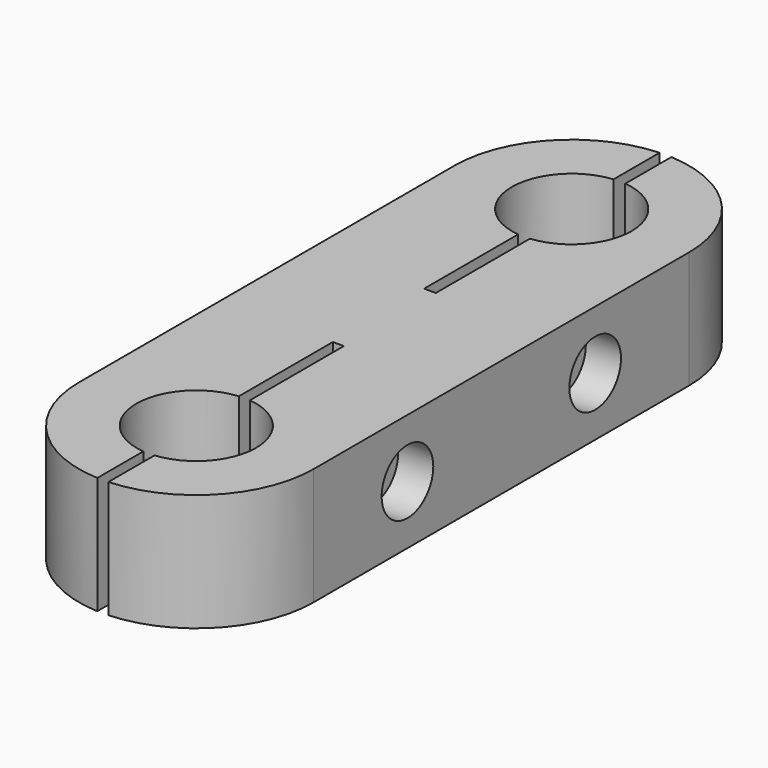
from build123d import *

# Parameters (mm, degrees)
F0_R     = 5.1
F1_DEPTH = 10
F2_R     = 1.5
F3_DEPTH = 25
F5_DEPTH = 25
F6_R     = 2.75
F6_R_2   = 1.5
F7_DEPTH = 3
F8_R     = 1.5
F9_DEPTH = 2


# Not quite as in the source:
# - a feature names something its author has since deleted; it is built from what else it names


with BuildPart() as f1:
    # F0 (on Top) → F1 (new body)
    with BuildSketch(Plane.XY):
        with BuildLine():
            ThreePointArc((-10, 0), (0, -10), (10, 0))
            ThreePointArc((10, 0), (0, 10), (-10, 0))
        make_face()
        Circle(F0_R, mode=Mode.SUBTRACT)
        with BuildLine():
            Line((10, -40), (10, 0))
            ThreePointArc((10, 0), (0, -10), (-10, 0))
            Line((-10, 0), (-10, -40))
            ThreePointArc((-10, -40), (0, -30), (10, -40))
        make_face()
        with BuildLine():
            ThreePointArc((-10, -40), (0, -50), (10, -40))
            ThreePointArc((10, -40), (0, -30), (-10, -40))
        make_face()
        with Locations((0, -40)):
            Circle(F0_R, mode=Mode.SUBTRACT)
    extrude(amount=F1_DEPTH)

    # F2 (on face) → F3 (cut)
    with BuildSketch(Plane.YZ.offset(10)):
        with Locations((-30, 5)):
            Circle(F2_R)
        with Locations((-10, 5)):
            Circle(F2_R)
    extrude(amount=-F3_DEPTH, mode=Mode.SUBTRACT)

    # F4 (on face) → F5 (cut)
    with BuildSketch(Plane.XY.offset(10)):
        with BuildLine():
            ThreePointArc((0.5, 9.9874921777), (0, 10), (-0.5, 9.9874921777))
            Line((-0.5, 9.9874921777), (-0.5, 5.0754310162))
            ThreePointArc((-0.5, 5.0754310162), (0, 5.1), (0.5, 5.0754310162))
            Line((0.5, 5.0754310162), (0.5, 9.9874921777))
        make_face()
        with BuildLine():
            ThreePointArc((0.5, -5.0754310162), (0, -5.1), (-0.5, -5.0754310162))
            Line((-0.5, -5.0754310162), (-0.5, -15.1))
            Line((-0.5, -15.1), (0.5, -15.1))
            Line((0.5, -15.1), (0.5, -5.0754310162))
        make_face()
        with BuildLine():
            Line((-0.439394009, -45.0810365975), (-0.439394009, -49.9903419814))
            ThreePointArc((-0.439394009, -49.9903419814), (0.0303364777, -49.9999539848), (0.5, -49.9874921777))
            Line((0.5, -49.9874921777), (0.5, -45.0754310162))
            ThreePointArc((0.5, -45.0754310162), (0.0304323376, -45.0999092024), (-0.439394009, -45.0810365975))
        make_face()
        with BuildLine():
            Line((-0.439394009, -24.9), (-0.439394009, -34.9189634025))
            ThreePointArc((-0.439394009, -34.9189634025), (0.0304323376, -34.9000907976), (0.5, -34.9245689838))
            Line((0.5, -34.9245689838), (0.5, -24.9))
            Line((0.5, -24.9), (-0.439394009, -24.9))
        make_face()
    extrude(amount=-F5_DEPTH, mode=Mode.SUBTRACT)

    # F6 (on face) → F7 (cut)
    with BuildSketch(Plane.YZ.offset(10)):
        with Locations((-30, 5)):
            Circle(F6_R)
        with Locations((-30, 5)):
            Circle(F6_R_2, mode=Mode.SUBTRACT)
        with Locations((-10, 5)):
            Circle(F6_R)
        with Locations((-10, 5)):
            Circle(F6_R_2, mode=Mode.SUBTRACT)
    extrude(amount=-F7_DEPTH, mode=Mode.SUBTRACT)

    # F8 (on face) → F9 (cut)
    with BuildSketch(Plane(origin=(-10, 0, 0), x_dir=(0, -1, 0), z_dir=(-1, 0, 0))):
        Polygon((8.4122867597, 2.25), (11.5877132403, 2.25), (13.1754264805, 5), (11.5877132403, 7.75), (8.4122867597, 7.75), (6.8245735195, 5), align=None)
        with Locations((10, 5)):
            Circle(F8_R, mode=Mode.SUBTRACT)
        Polygon((28.4122867597, 2.25), (31.5877132403, 2.25), (33.1754264805, 5), (31.5877132403, 7.75), (28.4122867597, 7.75), (26.8245735195, 5), align=None)
        with Locations((30, 5)):
            Circle(F8_R, mode=Mode.SUBTRACT)
    extrude(amount=-F9_DEPTH, mode=Mode.SUBTRACT)


solid = f1.part
